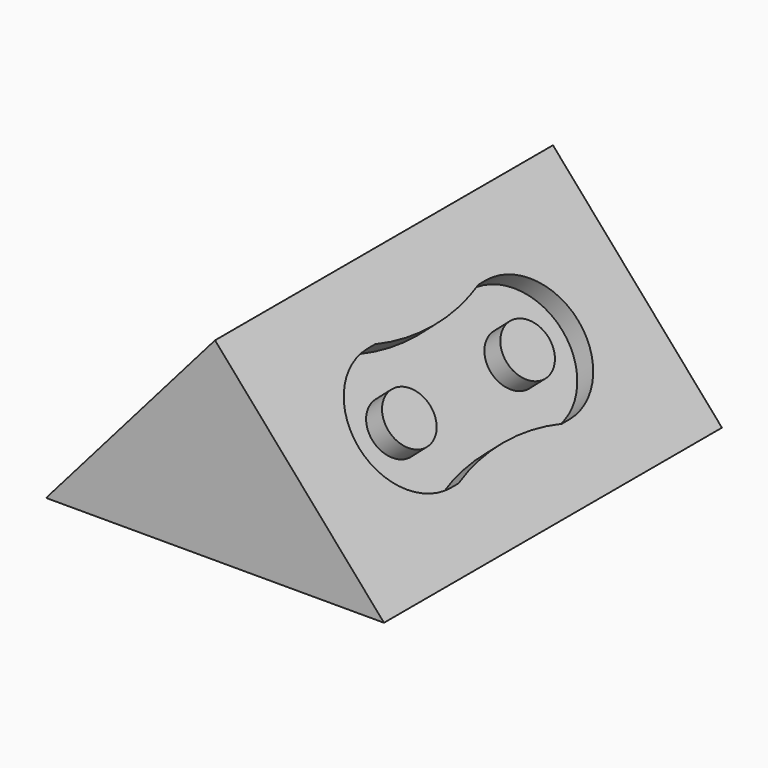
from build123d import *

# Parameters (mm, degrees)
F1_DEPTH = 254
F2_R     = 15.875
F3_DEPTH = 12.7


# Not quite as in the source:
# - a pattern or mirror of a feature is missing from the dataset's text; its kind, count and spacing are read off the source's solid


with BuildPart() as f1:
    # F0 (on Front) → F1 (new body)
    with BuildSketch(Plane.XZ):
        Polygon((101.6, 116.5001839399), (0, 0), (203.2, 0), align=None)
    extrude(amount=F1_DEPTH)

    # F2 (on face) → F3 (cut)
    with BuildSketch(Plane(origin=(115.4177397592, 0, 100.6559986685), x_dir=(0, 1, 0), z_dir=(0.7536582036, 0, 0.6572665458))):
        with BuildLine():
            Line((-165.875079947, -18.1667619065), (-171.45, -18.1667619065))
            ThreePointArc((-171.45, -18.1667619065), (-209.55, -56.2667619065), (-171.45, -94.3667619065))
            Line((-171.45, -94.3667619065), (-165.875079947, -94.3667619065))
            ThreePointArc((-165.875079947, -94.3667619065), (-127, -88.270559031), (-88.124920053, -94.3667619065))
            Line((-88.124920053, -94.3667619065), (-82.55, -94.3667619065))
            ThreePointArc((-82.55, -94.3667619065), (-44.45, -56.2667619065), (-82.55, -18.1667619065))
            Line((-82.55, -18.1667619065), (-88.124920053, -18.1667619065))
            ThreePointArc((-88.124920053, -18.1667619065), (-127, -24.262964782), (-165.875079947, -18.1667619065))
        make_face()
        with Locations((-171.45, -56.2667619065)):
            Circle(F2_R, mode=Mode.SUBTRACT)
        with Locations((-82.55, -56.2667619065)):
            Circle(F2_R, mode=Mode.SUBTRACT)
    f3 = extrude(amount=-F3_DEPTH, mode=Mode.SUBTRACT)

    # F3_copies: F3 across plane
    add(f3.mirror(Plane(origin=(101.6, 0, 0), x_dir=(0, 0, -1), z_dir=(-1, 0, 0))), mode=Mode.SUBTRACT)


solid = f1.part
